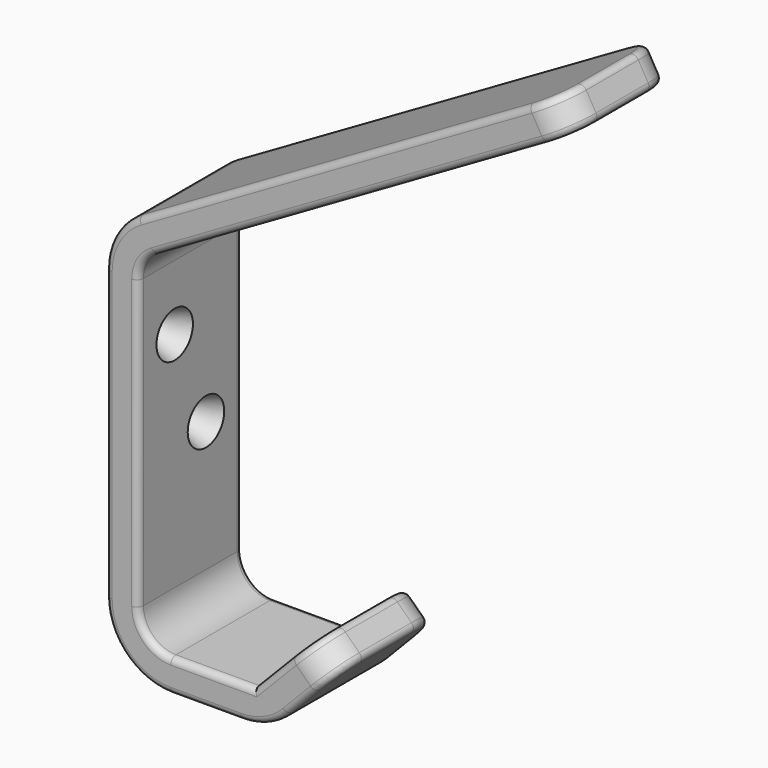
from build123d import *

# Parameters (mm, degrees)
F1_DEPTH        = 20
F2_R            = 10
F3_R            = 10
F5_R            = 5
F6_R            = 5
F7_R            = 5
F8_R            = 5
F9_R            = 5
F10_R           = 5
F11_R           = 1
F12_R           = 1
F13_R           = 1
F15_D           = 4
F15_CSINK_D     = 7
F15_CSINK_ANGLE = 45
F17_D           = 4
F17_CSINK_D     = 7
F17_CSINK_ANGLE = 45


# Not quite as in the source:
# - two fillets or chamfers of one size are made in one step


with BuildPart() as f1:
    # F0 (on Front) → F1 (new body)
    with BuildSketch(Plane.XZ):
        Polygon((-11.9194036352, -14.2478547741), (13.0805963648, -14.2478547741), (23.7375380173, -3.1786129853), (20.1516641766, 0.305853803), (10.8681305885, -9.2478547741), (-6.9194036352, -9.2478547741), (-6.9194036352, 42.86539388), (59.8626286675, 81.422018207), (57.3626286675, 85.7521452259), (-11.9194036352, 45.7521452259), align=None)
    extrude(amount=F1_DEPTH)

    # F2
    f2_edges = [f1.edges().sort_by_distance(p)[0] for p in [
        (-11.919404, -10, -14.247855),
    ]]
    fillet(f2_edges, radius=F2_R)

    # F3
    f3_edges = [f1.edges().sort_by_distance(p)[0] for p in [
        (-11.919404, -10, 45.752145),
        (13.080596, -10, -14.247855),
    ]]
    fillet(f3_edges, radius=F3_R)

    # F5
    f5_edges = [f1.edges().sort_by_distance(p)[0] for p in [
        (-6.919404, -10, -9.247855),
    ]]
    fillet(f5_edges, radius=F5_R)

    # F6
    f6_edges = [f1.edges().sort_by_distance(p)[0] for p in [
        (-6.919404, -10, 42.865394),
    ]]
    fillet(f6_edges, radius=F6_R)

    # F7
    f7_edges = [f1.edges().sort_by_distance(p)[0] for p in [
        (21.944601, -20, -1.43638),
    ]]
    fillet(f7_edges, radius=F7_R)

    # F8
    f8_edges = [f1.edges().sort_by_distance(p)[0] for p in [
        (21.944601, 0, -1.43638),
    ]]
    fillet(f8_edges, radius=F8_R)

    # F9
    f9_edges = [f1.edges().sort_by_distance(p)[0] for p in [
        (58.612629, -20, 83.587082),
    ]]
    fillet(f9_edges, radius=F9_R)

    # F10
    f10_edges = [f1.edges().sort_by_distance(p)[0] for p in [
        (58.612629, 0, 83.587082),
    ]]
    fillet(f10_edges, radius=F10_R)

    # F11
    f11_edges = [f1.edges().sort_by_distance(p)[0] for p in [
        (25.556549, -20, 61.615394),
    ]]
    fillet(f11_edges, radius=F11_R)

    # F12
    f12_edges = [f1.edges().sort_by_distance(p)[0] for p in [
        (18.150256, -20, -8.982058),
    ]]
    fillet(f12_edges, radius=F12_R)

    # F13
    f13_edges = [f1.edges().sort_by_distance(p)[0] for p in [
        (13.767664, -20, -6.263937),
        (13.767664, 0, -6.263937),
        (19.131087, -1.464466, -0.744424),
        (19.131087, -18.535534, -0.744424),
        (20.151664, -10, 0.305854),
    ]]
    fillet(f13_edges, radius=F13_R)

    # F15 (through all)
    with Locations(Plane.YZ.offset(-6.9194036352)):
        with Locations((-13, 29.978642534)):
            CounterSinkHole(F15_D / 2, F15_CSINK_D / 2, counter_sink_angle=F15_CSINK_ANGLE)

    # F17 (through all)
    with Locations(Plane.YZ.offset(-6.9194036352)):
        with Locations((-7, 15.7521452259)):
            CounterSinkHole(F17_D / 2, F17_CSINK_D / 2, counter_sink_angle=F17_CSINK_ANGLE)


solid = f1.part
